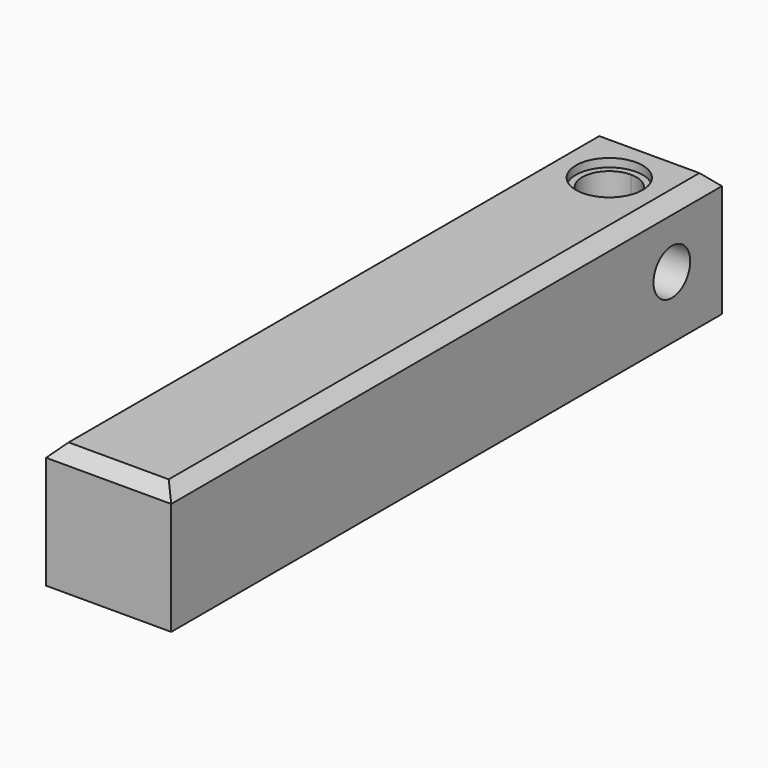
from build123d import *

# Parameters (mm, degrees)
F0_W      = 30
F0_H      = 30
F1_DEPTH  = 165
F3_DEPTH  = 30
F4_R      = 5.5
F5_DEPTH  = 12.3
F6_R      = 8
F6_R_2    = 6.5
F7_DEPTH  = 2
F8_SIZE   = 3
F10_DEPTH = 25


# Not quite as in the source:
# - a pattern or mirror of a feature is missing from the dataset's text; its kind, count and spacing are read off the source's solid


with BuildPart() as f1:
    # F0 (on Front) → F1 (new body)
    with BuildSketch(Plane.XZ):
        Rectangle(F0_W, F0_H)
    extrude(amount=F1_DEPTH)

    # F2 (on face) → F3 (cut)
    with BuildSketch(Plane.XY.offset(15)):
        with BuildLine():
            ThreePointArc((0, -8.5), (-4.5961940777, -19.5961940777), (6.5, -15))
            ThreePointArc((6.5, -15), (4.5961940777, -10.4038059223), (0, -8.5))
        make_face()
    extrude(amount=-F3_DEPTH, mode=Mode.SUBTRACT)

    # F4 (on face) → F5 (cut)
    with BuildSketch(Plane.YZ.offset(15)):
        with Locations((-15, 0)):
            Circle(F4_R)
    extrude(amount=-F5_DEPTH, mode=Mode.SUBTRACT)

    # F6 (on face) → F7 (cut)
    with BuildSketch(Plane.XY.offset(15)):
        with Locations((0, -15)):
            Circle(F6_R)
        with Locations((0, -15)):
            Circle(F6_R_2, mode=Mode.SUBTRACT)
        with Locations((0, -15)):
            Circle(F6_R_2)
    f7 = extrude(amount=-F7_DEPTH, mode=Mode.SUBTRACT)

    # F7_copies: F7 across plane
    add(f7.mirror(Plane(origin=(0, 0, 0), x_dir=(-1, 0, 0), z_dir=(0, 0, -1))), mode=Mode.SUBTRACT)

    # F8
    f8_edges = [f1.edges().sort_by_distance(p)[0] for p in [
        (15, -82.5, 15),
        (0, 0, 15),
        (-15, -82.5, 15),
        (0, -165, 15),
    ]]
    chamfer(f8_edges, length=F8_SIZE)

    # F9 (on face) → F10 (cut)
    with BuildSketch(Plane(origin=(0, 0, -15), x_dir=(1, 0, 0), z_dir=(0, 0, -1))):
        with BuildLine():
            ThreePointArc((0, 90.5), (-4, 86.5), (0, 82.5))
            Line((0, 82.5), (0, 86.5))
            Line((0, 86.5), (0, 90.5))
        make_face()
        with BuildLine():
            Line((0, 86.5), (0, 82.5))
            ThreePointArc((0, 82.5), (2.8284271247, 83.6715728753), (4, 86.5))
            ThreePointArc((4, 86.5), (2.8284271247, 89.3284271247), (0, 90.5))
            Line((0, 90.5), (0, 86.5))
        make_face()
        with BuildLine():
            ThreePointArc((4, 156.5), (-2.8284271247, 159.3284271247), (0, 152.5))
            ThreePointArc((0, 152.5), (2.8284271247, 153.6715728753), (4, 156.5))
        make_face()
    extrude(amount=-F10_DEPTH, mode=Mode.SUBTRACT)


solid = f1.part
